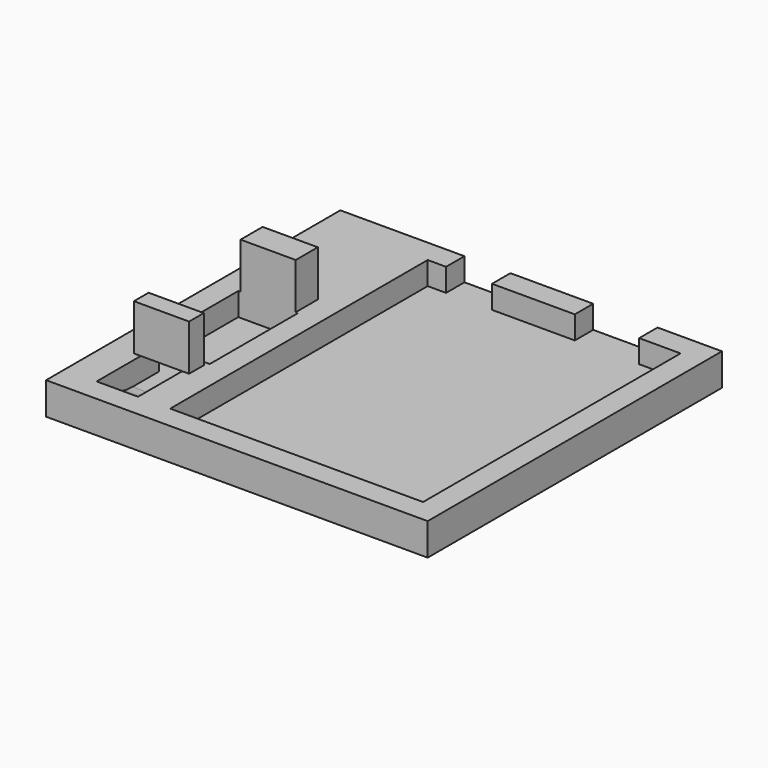
from build123d import *

# Parameters (mm, degrees)
F0_W         = 13
F0_H         = 24
F1_DEPTH     = 5
F0_W_2       = 18
F0_H_2       = 5
F2_W         = 83
F2_H         = 80
F3_DEPTH     = 2
F4_W         = 9
F4_H         = 17
F5_DEPTH     = 5
F6_W         = 12
F6_H         = 6
F7_DEPTH     = 10
F8_W         = 12
F8_H         = 4
F9_DEPTH     = 10
F10_T1_DEPTH = 9


# Not quite as in the source:
# - a fillet or chamfer that OpenCascade refuses, or shapes differently, is made with other operations: its cross-section is extruded or revolved along the edge and cut away or added


with BuildPart() as f1:
    # F0 (on Top) → F1 (new body)
    with BuildSketch(Plane.XY):
        Polygon((-19.7103468106, 42.4778270721), (-46.7103468106, 42.4778270721), (-46.7103468106, -37.5221729279), (36.2896531894, -37.5221729279), (36.2896531894, 42.4778270721), (22.2896531894, 42.4778270721), (22.2896531894, 37.4778270721), (31.2896531894, 37.4778270721), (31.2896531894, -32.5221729279), (-23.7103468106, -32.5221729279), (-23.7103468106, 37.4778270721), (-19.7103468106, 37.4778270721), align=None)
        with Locations((-35.2103468106, -3.5221729279)):
            Rectangle(F0_W, F0_H, mode=Mode.SUBTRACT)
    extrude(amount=F1_DEPTH)



with BuildPart() as f1b:
    # F0 (on Top) → F1, piece 2 (new body)
    with BuildSketch(Plane.XY):
        with Locations((-0.7103468106, 39.9778270721)):
            Rectangle(F0_W_2, F0_H_2)
    extrude(amount=F1_DEPTH)


with BuildPart() as f1_1:
    add(f1.part)

    add(f1b.part)  # F3 merges F1b
    # F2 (on face) → F3 (join)
    with BuildSketch(Plane(origin=(0, 0, 0), x_dir=(1, 0, 0), z_dir=(0, 0, -1))):
        with Locations((-5.2103468106, -2.4778270721)):
            Rectangle(F2_W, F2_H)
    extrude(amount=F3_DEPTH)

    # F4 (on face) → F5 (cut)
    with BuildSketch(Plane.XY.offset(5)):
        with Locations((-35.2103468106, -24.0221729279)):
            Rectangle(F4_W, F4_H)
    extrude(amount=-F5_DEPTH, mode=Mode.SUBTRACT)

    # F6 (on face) → F7 (join)
    with BuildSketch(Plane.XY.offset(5)):
        with Locations((-35.2103468106, 11.4778270721)):
            Rectangle(F6_W, F6_H)
    extrude(amount=F7_DEPTH)

    # F8 (on face) → F9 (join)
    with BuildSketch(Plane.XY.offset(5)):
        with Locations((-35.2103468106, -18.5221729279)):
            Rectangle(F8_W, F8_H)
    extrude(amount=F9_DEPTH)

    # F10: fillet of radius 12 on 1 edges, made by hand

    # F10_s2 → F10_t1 (join)
    with BuildSketch(Plane.YZ.offset(-39.7103468106)):
        with BuildLine():
            ThreePointArc((-32.5221729279, 5), (-28.2526041581, 1.322921748), (-22.775378583, 0))
            Line((-22.775378583, 0), (-32.5221729279, 0))
            Line((-32.5221729279, 0), (-32.5221729279, 5))
        make_face()
    extrude(amount=F10_T1_DEPTH)


solid = f1_1.part
